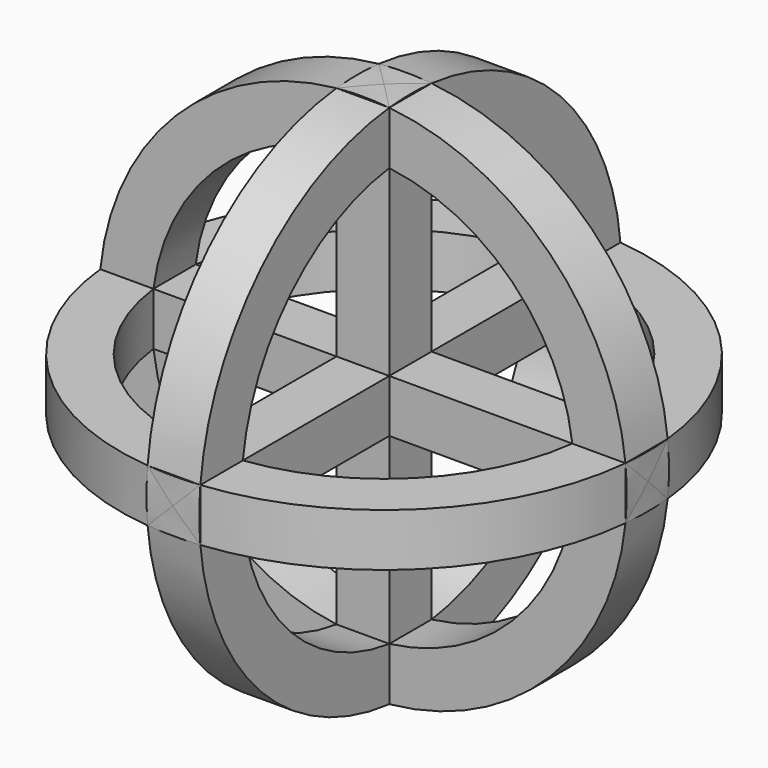
from build123d import *

# Parameters (mm, degrees)
F0_R          = 12.7
F1_DEPTH      = 1.27
F1_DEPTH_BACK = 1.27
F0_W          = 2.54
F0_H          = 2.54
F2_DEPTH      = 10.16
F2_DEPTH_BACK = 10.16
F3_DEPTH      = 1.27
F3_DEPTH_BACK = 1.27
F4_DEPTH      = 1.27
F4_DEPTH_BACK = 1.27
F5_DEPTH      = 1.27
F5_DEPTH_BACK = 1.27
F6_DEPTH      = 1.27
F6_DEPTH_BACK = 1.27


# Not quite as in the source:
# - a feature of the source that left no trace in its solid (it failed there, or was rolled back) is left out
# - a pattern or mirror of a feature is missing from the dataset's text; its kind, count and spacing are read off the source's solid


with BuildPart() as f1:
    # F0 (on Right) → F1 (new body, two sides)
    with BuildSketch(Plane.YZ) as f1_sk:
        Circle(F0_R)
        with BuildLine():
            ThreePointArc((-10.0803124952, 1.27), (-7.1842048969, 7.1842048969), (-1.27, 10.0803124952))
            ThreePointArc((-1.27, 10.0803124952), (0, 10.16), (1.27, 10.0803124952))
            ThreePointArc((1.27, 10.0803124952), (7.1842048969, 7.1842048969), (10.0803124952, 1.27))
            ThreePointArc((10.0803124952, 1.27), (10.1400585538, 0.6362487914), (10.16, 0))
            ThreePointArc((10.16, 0), (10.1400585538, -0.6362487914), (10.0803124952, -1.27))
            ThreePointArc((10.0803124952, -1.27), (7.1842048969, -7.1842048969), (1.27, -10.0803124952))
            ThreePointArc((1.27, -10.0803124952), (0, -10.16), (-1.27, -10.0803124952))
            ThreePointArc((-1.27, -10.0803124952), (-7.1842048969, -7.1842048969), (-10.0803124952, -1.27))
            ThreePointArc((-10.0803124952, -1.27), (-10.16, 0), (-10.0803124952, 1.27))
        make_face(mode=Mode.SUBTRACT)
    extrude(amount=F1_DEPTH)
    extrude(f1_sk.sketch, amount=-F1_DEPTH_BACK)

    # F1_copies: F1 across plane


with BuildPart() as f1_1:
    add(f1.part)
    add(f1.part.mirror(Plane(origin=(0, 0, 0), x_dir=(0.7071067812, 0, -0.7071067812), z_dir=(0.7071067812, 0, 0.7071067812))))

    # F1_copies1: F1 across plane


with BuildPart() as f1_2:
    add(f1_1.part)
    add(f1_1.part.mirror(Plane(origin=(0, 0, 0), x_dir=(-0.7071067812, 0.7071067812, 0), z_dir=(-0.7071067812, -0.7071067812, 0))))

    # F0 (on Right) → F2 (join, two sides)
    with BuildSketch(Plane.YZ) as f2_sk:
        Rectangle(F0_W, F0_H)
    extrude(amount=F2_DEPTH)
    extrude(f2_sk.sketch, amount=-F2_DEPTH_BACK)

    # F0 (on Right) → F3 (join, two sides)
    with BuildSketch(Plane.YZ) as f3_sk:
        with BuildLine():
            Line((1.27, -1.27), (-1.27, -1.27))
            Line((-1.27, -1.27), (-1.27, -10.0803124952))
            ThreePointArc((-1.27, -10.0803124952), (0, -10.16), (1.27, -10.0803124952))
            Line((1.27, -10.0803124952), (1.27, -1.27))
        make_face()
    extrude(amount=F3_DEPTH)
    extrude(f3_sk.sketch, amount=-F3_DEPTH_BACK)

    # F0 (on Right) → F4 (join, two sides)
    with BuildSketch(Plane.YZ) as f4_sk:
        with BuildLine():
            Line((10.0803124952, 1.27), (1.27, 1.27))
            Line((1.27, 1.27), (1.27, -1.27))
            Line((1.27, -1.27), (10.0803124952, -1.27))
            ThreePointArc((10.0803124952, -1.27), (10.1400585538, -0.6362487914), (10.16, 0))
            ThreePointArc((10.16, 0), (10.1400585538, 0.6362487914), (10.0803124952, 1.27))
        make_face()
    extrude(amount=F4_DEPTH)
    extrude(f4_sk.sketch, amount=-F4_DEPTH_BACK)

    # F0 (on Right) → F5 (join, two sides)
    with BuildSketch(Plane.YZ) as f5_sk:
        with BuildLine():
            Line((-1.27, -1.27), (-1.27, 1.27))
            Line((-1.27, 1.27), (-10.0803124952, 1.27))
            ThreePointArc((-10.0803124952, 1.27), (-10.16, 0), (-10.0803124952, -1.27))
            Line((-10.0803124952, -1.27), (-1.27, -1.27))
        make_face()
    extrude(amount=F5_DEPTH)
    extrude(f5_sk.sketch, amount=-F5_DEPTH_BACK)

    # F0 (on Right) → F6 (join, two sides)
    with BuildSketch(Plane.YZ) as f6_sk:
        with BuildLine():
            Line((-1.27, 10.0803124952), (-1.27, 1.27))
            Line((-1.27, 1.27), (1.27, 1.27))
            Line((1.27, 1.27), (1.27, 10.0803124952))
            ThreePointArc((1.27, 10.0803124952), (0, 10.16), (-1.27, 10.0803124952))
        make_face()
    extrude(amount=F6_DEPTH)
    extrude(f6_sk.sketch, amount=-F6_DEPTH_BACK)


solid = f1_2.part
